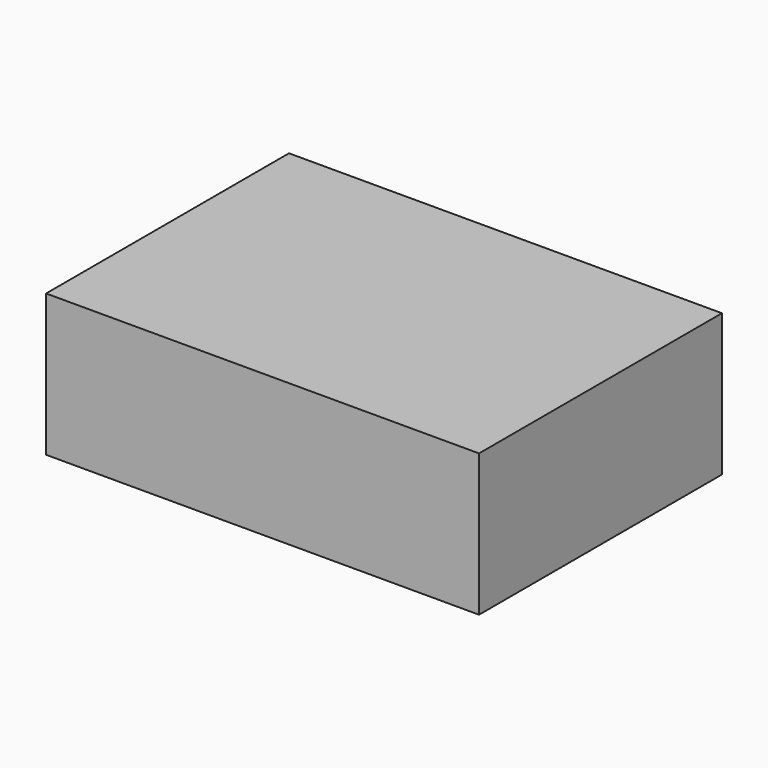
from build123d import *

# Parameters (mm, degrees)
F0_W     = 77.4215683341
F0_H     = 54.293114692
F1_DEPTH = 25.4


# Not quite as in the source:
# - the program builds the solid bodies; features that only make, move or delete a surface that nothing else refers to are left out


with BuildPart() as f1:
    # F0 (on Top) → F1 (new body)
    with BuildSketch(Plane.XY):
        with Locations((38.7107841671, -27.146557346)):
            Rectangle(F0_W, F0_H)
    extrude(amount=F1_DEPTH)


solid = f1.part
